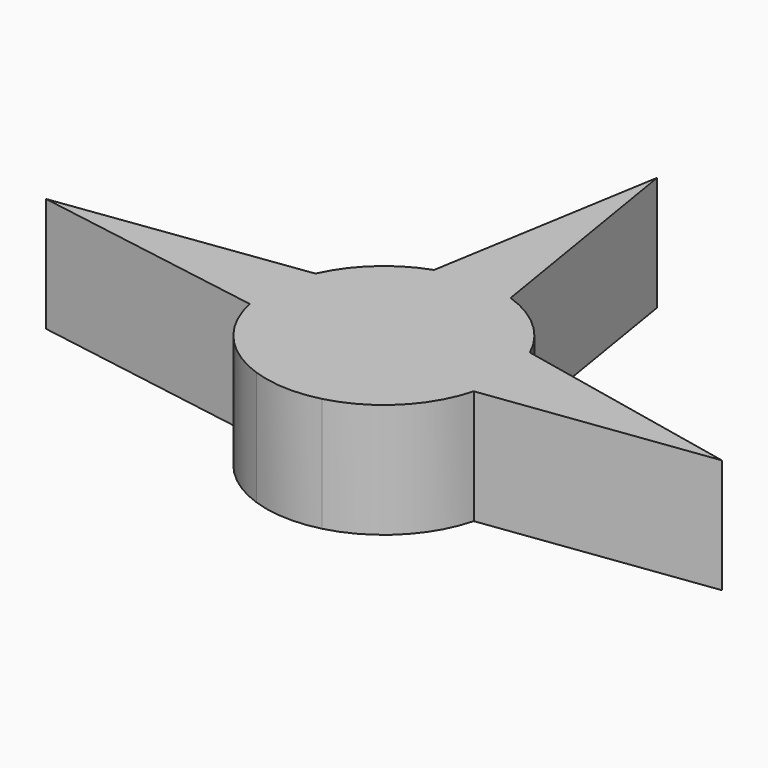
from build123d import *

# Parameters (mm, degrees)
F1_DEPTH = 25


with BuildPart() as f1:
    # F0 (on Top) → F1 (new body)
    with BuildSketch(Plane.XY):
        with BuildLine():
            ThreePointArc((24.8701038765, -6.5218529704), (25.4999256036, -3.2879214113), (25.7110216249, 0))
            ThreePointArc((25.7110216249, 0), (25.1255094172, 5.4557684631), (23.3956403104, 10.6630505701))
            ThreePointArc((23.3956403104, 10.6630505701), (17.2285716474, 19.0848880527), (8.2217665775, 24.3610177813))
            ThreePointArc((8.2217665775, 24.3610177813), (-0.1258474148, 25.7107136311), (-8.459848903, 24.2793655093))
            ThreePointArc((-8.459848903, 24.2793655093), (-17.3538464261, 18.9710476046), (-23.4315262789, 10.5839599978))
            ThreePointArc((-23.4315262789, 10.5839599978), (-25.5543270236, 2.8342553459), (-25.1812828872, -5.1922658973))
            ThreePointArc((-25.1812828872, -5.1922658973), (-19.3520995784, -16.9278727223), (-8.4963727751, -24.2666083881))
            ThreePointArc((-8.4963727751, -24.2666083881), (-1.0796944371, -25.6883415758), (6.430127649, -24.8939770108))
            ThreePointArc((6.430127649, -24.8939770108), (18.146896672, -18.2139170463), (24.8701038765, -6.5218529704))
        make_face()
        with BuildLine():
            ThreePointArc((23.3956403104, 10.6630505701), (25.1255094172, 5.4557684631), (25.7110216249, 0))
            ThreePointArc((25.7110216249, 0), (25.4999256036, -3.2879214113), (24.8701038765, -6.5218529704))
            Line((24.8701038765, -6.5218529704), (73.9221572876, 0))
            Line((73.9221572876, 0), (23.3956403104, 10.6630505701))
        make_face()
        with BuildLine():
            ThreePointArc((-8.459848903, 24.2793655093), (-0.1258474148, 25.7107136311), (8.2217665775, 24.3610177813))
            Line((8.2217665775, 24.3610177813), (0, 74.7051164508))
            Line((0, 74.7051164508), (-8.459848903, 24.2793655093))
        make_face()
        with BuildLine():
            ThreePointArc((-25.1812828872, -5.1922658973), (-25.5543270236, 2.8342553459), (-23.4315262789, 10.5839599978))
            Line((-23.4315262789, 10.5839599978), (-76.5798836946, 3.3824506681))
            Line((-76.5798836946, 3.3824506681), (-25.1812828872, -5.1922658973))
        make_face()
    extrude(amount=F1_DEPTH)


solid = f1.part
